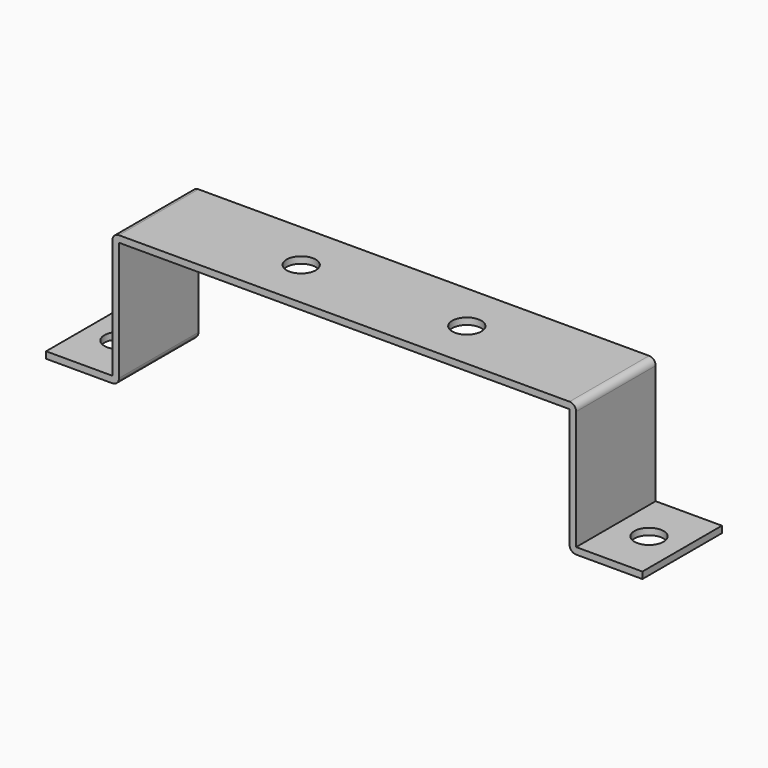
from build123d import *

# Parameters (mm, degrees)
F1_DEPTH = 30
F2_R     = 4.4
F3_R     = 4.4
F4_DEPTH = 25
F5_R     = 2
F6_R     = 2


# Not quite as in the source:
# - a feature names something its author has since deleted; it is built from what else it names


with BuildPart() as f1:
    # F0 (on Front) → F1 (new body)
    with BuildSketch(Plane.XZ):
        Polygon((90, -1), (90, 1), (70, 1), (70, 39), (-70, 39), (-70, 1), (-90, 1), (-90, -1), (-68, -1), (-68, 37), (68, 37), (68, -1), align=None)
    extrude(amount=F1_DEPTH)

    # F2 (on face) + F3 (on face) → F4 (cut)
    with BuildSketch(Plane.XY.offset(1)):
        with Locations((-80, -15)):
            Circle(F2_R)
        with Locations((80, -15)):
            Circle(F2_R)
    with BuildSketch(Plane.XY.offset(39)):
        with Locations((-25, -15)):
            Circle(F3_R)
        with Locations((25, -15)):
            Circle(F3_R)
    extrude(amount=-F4_DEPTH, mode=Mode.SUBTRACT)

    # F5
    f5_edges = [f1.edges().sort_by_distance(p)[0] for p in [
        (-70, -15, 39),
        (70, -15, 39),
    ]]
    fillet(f5_edges, radius=F5_R)

    # F6
    f6_edges = [f1.edges().sort_by_distance(p)[0] for p in [
        (68, -15, -1),
        (-68, -15, -1),
    ]]
    fillet(f6_edges, radius=F6_R)


solid = f1.part
